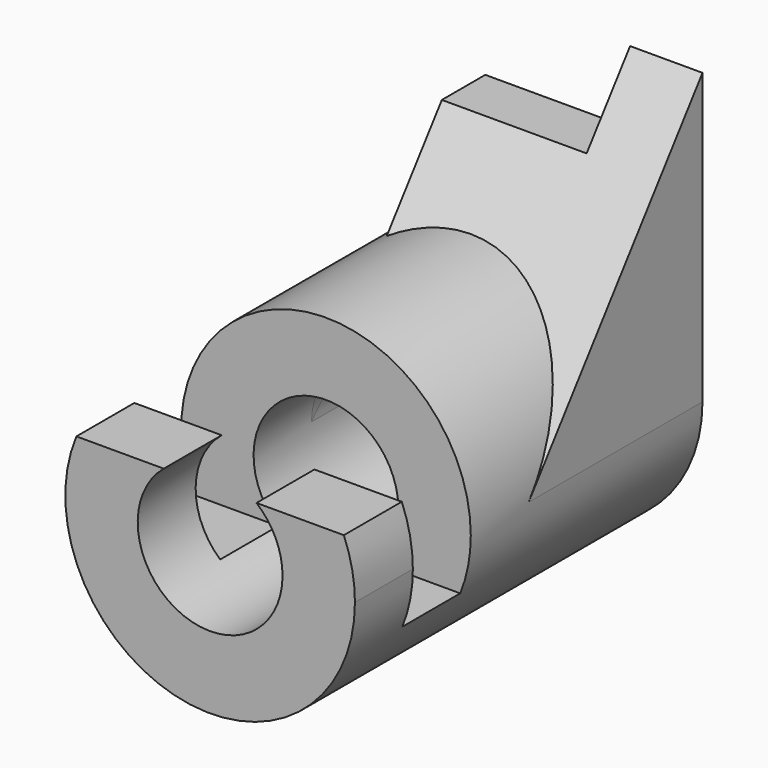
from build123d import *

# Parameters (mm, degrees)
F0_R          = 25.4
F0_R_2        = 12.7
F1_DEPTH      = 76.2
F3_DEPTH      = 12.7
F5_START      = -12.7
F5_DEPTH      = 12.7
F7_DEPTH      = 25.4
F7_DEPTH_BACK = 12.7
F9_DEPTH      = 38.1
F10_W         = 25.4
F10_H         = 12.7
F11_DEPTH     = 25.4


with BuildPart() as f1:
    # F0 (on Front) → F1 (new body)
    with BuildSketch(Plane.XZ):
        Circle(F0_R)
        Circle(F0_R_2, mode=Mode.SUBTRACT)
    extrude(amount=-F1_DEPTH)

    # F2 (on face) → F3 (cut)
    with BuildSketch(Plane.XZ):
        with BuildLine():
            Line((8.1350766981, 9.7524626181), (23.4531335408, 9.7524626181))
            ThreePointArc((23.4531335408, 9.7524626181), (0, 25.4), (-23.4531335408, 9.7524626181))
            Line((-23.4531335408, 9.7524626181), (-8.1350766981, 9.7524626181))
            ThreePointArc((-8.1350766981, 9.7524626181), (0, 12.7), (8.1350766981, 9.7524626181))
        make_face()
    extrude(amount=-F3_DEPTH, mode=Mode.SUBTRACT)

    # F4 (on face) → F5 (cut)
    with BuildSketch(Plane.XZ.offset(F5_START)):
        with BuildLine():
            Line((23.5464301965, -9.525), (38.1, -9.525))
            Line((38.1, -9.525), (38.1, 25.4))
            Line((38.1, 25.4), (-38.1, 25.4))
            Line((-38.1, 25.4), (-38.1, -9.525))
            Line((-38.1, -9.525), (-23.5464301965, -9.525))
            ThreePointArc((-23.5464301965, -9.525), (-25.39970254, 0.1229263078), (-23.4531335408, 9.7524626181))
            Line((-23.4531335408, 9.7524626181), (-8.1350766981, 9.7524626181))
            ThreePointArc((-8.1350766981, 9.7524626181), (-12.698798549, 0.1746866087), (-8.4002604126, -9.525))
            Line((-8.4002604126, -9.525), (8.4002604126, -9.525))
            ThreePointArc((8.4002604126, -9.525), (11.5752604126, -5.2252604126), (12.7, 0))
            ThreePointArc((12.7, 0), (11.5022926859, 5.3839820735), (8.1350766981, 9.7524626181))
            Line((8.1350766981, 9.7524626181), (23.4531335408, 9.7524626181))
            ThreePointArc((23.4531335408, 9.7524626181), (24.908528579, 4.9724444724), (25.4, 0))
            ThreePointArc((25.4, 0), (24.9323016085, -4.8518384664), (23.5464301965, -9.525))
        make_face()
        with BuildLine():
            ThreePointArc((-23.4531335408, 9.7524626181), (-25.39970254, 0.1229263078), (-23.5464301965, -9.525))
            Line((-23.5464301965, -9.525), (-8.4002604126, -9.525))
            ThreePointArc((-8.4002604126, -9.525), (-12.698798549, 0.1746866087), (-8.1350766981, 9.7524626181))
            Line((-8.1350766981, 9.7524626181), (-23.4531335408, 9.7524626181))
        make_face()
        with BuildLine():
            Line((8.4002604126, -9.525), (23.5464301965, -9.525))
            ThreePointArc((23.5464301965, -9.525), (24.9323016085, -4.8518384664), (25.4, 0))
            ThreePointArc((25.4, 0), (24.908528579, 4.9724444724), (23.4531335408, 9.7524626181))
            Line((23.4531335408, 9.7524626181), (8.1350766981, 9.7524626181))
            ThreePointArc((8.1350766981, 9.7524626181), (11.5022926859, 5.3839820735), (12.7, 0))
            ThreePointArc((12.7, 0), (11.5752604126, -5.2252604126), (8.4002604126, -9.525))
        make_face()
    extrude(amount=-F5_DEPTH, mode=Mode.SUBTRACT)

    # F6 (on Right) → F7 (join, two sides)
    with BuildSketch(Plane.YZ) as f7_sk:
        Polygon((38.1, 0), (76.2, 0), (76.2, 50.8), align=None)
    extrude(amount=F7_DEPTH)
    extrude(f7_sk.sketch, amount=-F7_DEPTH_BACK)

    # F8 (on face) → F9 (cut)
    with BuildSketch(Plane(origin=(0, 76.2, 0), x_dir=(-1, 0, 0), z_dir=(0, 1, 0))):
        with BuildLine():
            Line((-12.7, 0), (12.7, 0))
            ThreePointArc((12.7, 0), (0, 12.7), (-12.7, 0))
        make_face()
    extrude(amount=-F9_DEPTH, mode=Mode.SUBTRACT)

    # F10 (on face) → F11 (cut)
    with BuildSketch(Plane(origin=(0, 76.2, 0), x_dir=(-1, 0, 0), z_dir=(0, 1, 0))):
        with Locations((0, 44.45)):
            Rectangle(F10_W, F10_H)
    extrude(amount=-F11_DEPTH, mode=Mode.SUBTRACT)


solid = f1.part
